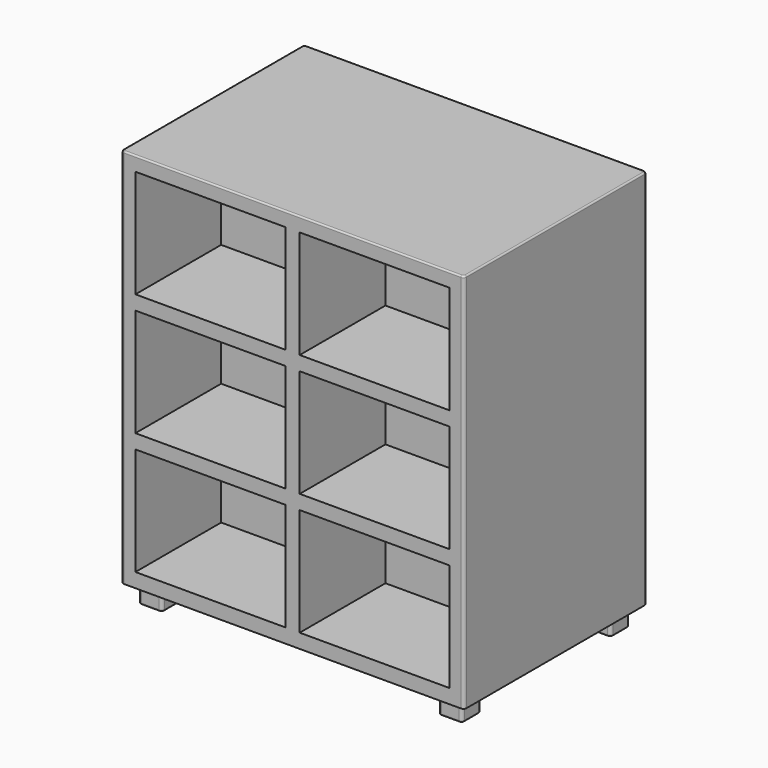
from build123d import *

# Parameters (mm, degrees)
F0_W     = 400.05
F0_H     = 287.8666666667
F1_DEPTH = 304.8
F2_DEPTH = 19.05
F3_W     = 63.5
F3_H     = 63.5
F4_DEPTH = 50.8
F5_SCALE = 0.0625
F6_R     = 0.508
F7_R     = 0.254


with BuildPart() as f1:
    # F0 (on Front) → F1 (new body, symmetric)
    with BuildSketch(Plane.XZ):
        Polygon((-457.2, 1066.8), (-457.2, 50.8), (-406.4, 50.8), (-355.6, 50.8), (355.6, 50.8), (406.4, 50.8), (457.2, 50.8), (457.2, 1066.8), align=None)
        with Locations((-219.075, 232.8333333333)):
            Rectangle(F0_W, F0_H, mode=Mode.SUBTRACT)
        with Locations((219.075, 232.8333333333)):
            Rectangle(F0_W, F0_H, mode=Mode.SUBTRACT)
        with Locations((-219.075, 558.8)):
            Rectangle(F0_W, F0_H, mode=Mode.SUBTRACT)
        with Locations((-219.075, 884.7666666667)):
            Rectangle(F0_W, F0_H, mode=Mode.SUBTRACT)
        with Locations((219.075, 558.8)):
            Rectangle(F0_W, F0_H, mode=Mode.SUBTRACT)
        with Locations((219.075, 884.7666666667)):
            Rectangle(F0_W, F0_H, mode=Mode.SUBTRACT)
    extrude(amount=F1_DEPTH, both=True)

    # F0 (on Front) → F2 (join, symmetric)
    with BuildSketch(Plane.XZ):
        with Locations((-219.075, 884.7666666667)):
            Rectangle(F0_W, F0_H)
        with Locations((219.075, 884.7666666667)):
            Rectangle(F0_W, F0_H)
        with Locations((219.075, 558.8)):
            Rectangle(F0_W, F0_H)
        with Locations((-219.075, 558.8)):
            Rectangle(F0_W, F0_H)
        with Locations((219.075, 232.8333333333)):
            Rectangle(F0_W, F0_H)
        with Locations((-219.075, 232.8333333333)):
            Rectangle(F0_W, F0_H)
    extrude(amount=F2_DEPTH, both=True)

    # F3 (on Top) → F4 (join, through all)
    with BuildSketch(Plane.XY):
        with Locations((-400.05, -247.65)):
            Rectangle(F3_W, F3_H)
        with Locations((400.05, -247.65)):
            Rectangle(F3_W, F3_H)
        with Locations((400.05, 247.65)):
            Rectangle(F3_W, F3_H)
        with Locations((-400.05, 247.65)):
            Rectangle(F3_W, F3_H)
    extrude(amount=F4_DEPTH)


with BuildPart() as f1_1:
    # F5: moved
    add(f1.part.scale(F5_SCALE))

    # F6
    f6_edges = [f1_1.edges().sort_by_distance(p)[0] for p in [
        (26.9875, 17.4625, 1.5875),
        (26.9875, 13.49375, 1.5875),
        (23.01875, 17.4625, 1.5875),
        (23.01875, 13.49375, 1.5875),
        (23.01875, -13.49375, 1.5875),
        (26.9875, -13.49375, 1.5875),
        (26.9875, -17.4625, 1.5875),
        (23.01875, -17.4625, 1.5875),
        (-23.01875, -17.4625, 1.5875),
        (-23.01875, -13.49375, 1.5875),
        (-26.9875, -17.4625, 1.5875),
        (-26.9875, -13.49375, 1.5875),
        (-23.01875, 17.4625, 1.5875),
        (-23.01875, 13.49375, 1.5875),
        (-26.9875, 13.49375, 1.5875),
        (-26.9875, 17.4625, 1.5875),
        (-28.575, 19.05, 34.925),
        (-28.575, -19.05, 34.925),
        (28.575, 19.05, 34.925),
        (28.575, -19.05, 34.925),
    ]]
    fillet(f6_edges, radius=F6_R)

    # F7
    f7_edges = [f1_1.edges().sort_by_distance(p)[0] for p in [
        (-28.575, 0, 66.675),
        (-26.9875, 15.478125, 0),
        (-25.003125, -13.49375, 0),
        (25.003125, -17.4625, 0),
        (25.003125, 13.49375, 0),
        (-25.003125, 17.4625, 3.175),
        (-23.16754, 17.31371, 3.175),
        (-26.83871, 17.31371, 3.175),
        (-23.01875, 15.478125, 3.175),
        (-26.9875, 15.478125, 3.175),
        (-23.16754, 13.64254, 3.175),
        (-26.83871, 13.64254, 3.175),
        (-25.003125, 13.49375, 3.175),
        (25.003125, 13.49375, 3.175),
        (23.16754, 13.64254, 3.175),
        (26.83871, 13.64254, 3.175),
        (23.01875, 15.478125, 3.175),
        (26.9875, 15.478125, 3.175),
        (23.16754, 17.31371, 3.175),
        (26.83871, 17.31371, 3.175),
        (25.003125, 17.4625, 3.175),
        (-23.01875, -15.478125, 3.175),
        (-23.16754, -17.31371, 3.175),
        (-23.16754, -13.64254, 3.175),
        (-25.003125, -17.4625, 3.175),
        (-25.003125, -13.49375, 3.175),
        (-26.83871, -17.31371, 3.175),
        (-26.83871, -13.64254, 3.175),
        (-26.9875, -15.478125, 3.175),
        (23.01875, -15.478125, 3.175),
        (23.16754, -13.64254, 3.175),
        (23.16754, -17.31371, 3.175),
        (25.003125, -13.49375, 3.175),
        (25.003125, -17.4625, 3.175),
        (26.83871, -13.64254, 3.175),
        (26.83871, -17.31371, 3.175),
        (26.9875, -15.478125, 3.175),
        (-28.42621, 18.90121, 66.675),
        (-28.42621, -18.90121, 66.675),
        (0, 19.05, 66.675),
        (28.42621, 18.90121, 66.675),
        (28.575, 0, 66.675),
        (28.42621, -18.90121, 66.675),
        (0, -19.05, 66.675),
        (-25.003125, 17.4625, 0),
        (-23.16754, 17.31371, 0),
        (-26.83871, 17.31371, 0),
        (-23.01875, 15.478125, 0),
        (-23.16754, 13.64254, 0),
        (-26.83871, 13.64254, 0),
        (-25.003125, 13.49375, 0),
        (23.16754, 13.64254, 0),
        (26.83871, 13.64254, 0),
        (23.01875, 15.478125, 0),
        (26.9875, 15.478125, 0),
        (23.16754, 17.31371, 0),
        (26.83871, 17.31371, 0),
        (25.003125, 17.4625, 0),
        (-23.01875, -15.478125, 0),
        (-23.16754, -17.31371, 0),
        (-23.16754, -13.64254, 0),
        (-25.003125, -17.4625, 0),
        (-26.83871, -17.31371, 0),
        (-26.83871, -13.64254, 0),
        (-26.9875, -15.478125, 0),
        (23.01875, -15.478125, 0),
        (23.16754, -13.64254, 0),
        (23.16754, -17.31371, 0),
        (25.003125, -13.49375, 0),
        (26.83871, -13.64254, 0),
        (26.83871, -17.31371, 0),
        (26.9875, -15.478125, 0),
    ]]
    fillet(f7_edges, radius=F7_R)


solid = f1_1.part
